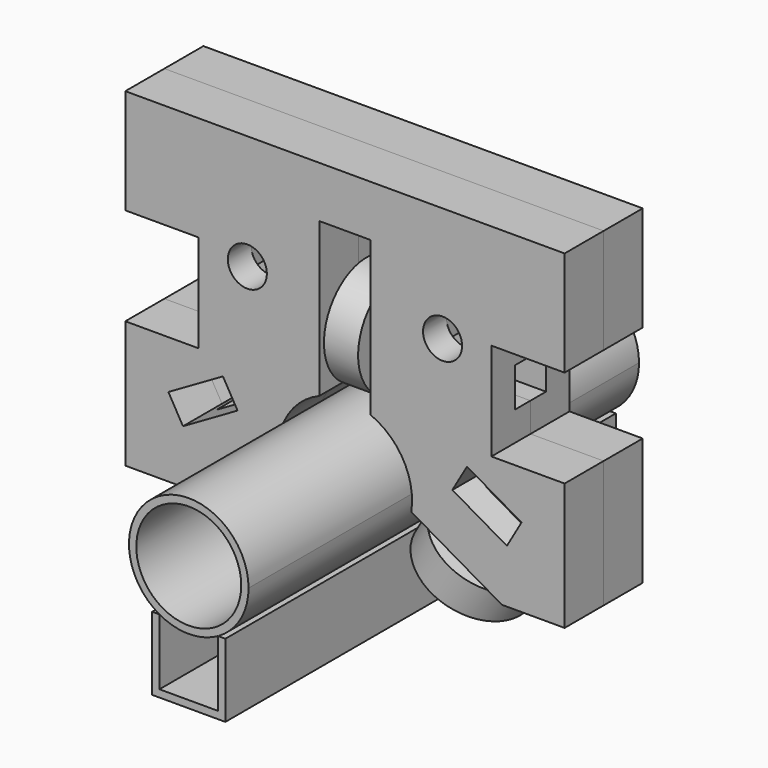
from build123d import *

# Parameters (mm, degrees)
F1_DEPTH = 50
F0_R     = 10.75
F2_R     = 11
F2_R_2   = 4
F3_DEPTH = 3.5
F5_COUNT = 3
F5_ANGLE = 240
F6_R     = 4
F7_DEPTH = 10
F9_DEPTH = 4


with BuildPart() as f1:
    # F0 (on Front) → F1 (new body, symmetric)
    with BuildSketch(Plane.XZ):
        Polygon((-6, -24.1800046816), (-6, -10.6800046816), (-7.5, -10.6800046816), (-7.5, -25.6800046816), (0, -25.6800046816), (7.5, -25.6800046816), (7.5, -10.6800046816), (6, -10.6800046816), (6, -24.1800046816), (0, -24.1800046816), align=None)
    extrude(amount=F1_DEPTH, both=True)


with BuildPart() as f1b:
    # F0 (on Front) → F1, piece 2 (new body, symmetric)
    with BuildSketch(Plane.XZ):
        with BuildLine():
            ThreePointArc((6, -10.6800046816), (10.5726652269, -6.1871843354), (12.25, 0))
            ThreePointArc((12.25, 0), (-6.1871843354, 10.5726652269), (-6, -10.6800046816))
            ThreePointArc((-6, -10.6800046816), (0, -12.25), (6, -10.6800046816))
        make_face()
        Circle(F0_R, mode=Mode.SUBTRACT)
    extrude(amount=F1_DEPTH, both=True)


with BuildPart() as f3:
    # F2 (on Right) → F3 (new body, symmetric)
    with BuildSketch(Plane.YZ):
        with Locations((0, 23.25)):
            Circle(F2_R)
        with Locations((0, 23.25)):
            Circle(F2_R_2, mode=Mode.SUBTRACT)
    extrude(amount=F3_DEPTH, both=True)


with BuildPart() as f5_1:
    # F5: instance of F3
    add(f3.part.rotate(Axis((0, 0, 0), (0, -1, 0)), 1 * F5_ANGLE / (F5_COUNT - 1)))


with BuildPart() as f5_2:
    # F5: instance of F3
    add(f3.part.rotate(Axis((0, 0, 0), (0, -1, 0)), 2 * F5_ANGLE / (F5_COUNT - 1)))


with BuildPart() as f7:
    # F6 (on Front) → F7 (new body)
    with BuildSketch(Plane.XZ):
        with BuildLine():
            ThreePointArc((5.25, 12.7082650271), (11.974631777, 6.7580096038), (13.5926495933, -2.0742172098))
            Line((13.5926495933, -2.0742172098), (32.1613700796, -12.7948729811))
            Line((32.1613700796, -12.7948729811), (45, -12.7948729811))
            Line((45, -12.7948729811), (45, 13.25))
            Line((45, 13.25), (30, 13.25))
            Line((30, 13.25), (30, 33.25))
            Line((30, 33.25), (45, 33.25))
            Line((45, 33.25), (45, 54.75))
            Line((45, 54.75), (0, 54.75))
            Line((0, 54.75), (-45, 54.75))
            Line((-45, 54.75), (-45, 33.25))
            Line((-45, 33.25), (-30, 33.25))
            Line((-30, 33.25), (-30, 13.25))
            Line((-30, 13.25), (-45, 13.25))
            Line((-45, 13.25), (-45, -12.7948729811))
            Line((-45, -12.7948729811), (-32.1613700796, -12.7948729811))
            Line((-32.1613700796, -12.7948729811), (-13.5926495933, -2.0742172098))
            ThreePointArc((-13.5926495933, -2.0742172098), (-11.974631777, 6.7580096038), (-5.25, 12.7082650271))
            Line((-5.25, 12.7082650271), (-5.25, 44.25))
            Line((-5.25, 44.25), (0, 44.25))
            Line((0, 44.25), (5.25, 44.25))
            Line((5.25, 44.25), (5.25, 12.7082650271))
        make_face()
        Polygon((-36.1776532222, 3.3615334795), (-25.0059255134, 9.8115334795), (-22.0059255134, 4.6153810568), (-33.1776532222, -1.8346189432), align=None, mode=Mode.SUBTRACT)
        Polygon((33.1776532222, -1.8346189432), (22.0059255134, 4.6153810568), (25.0059255134, 9.8115334795), (36.1776532222, 3.3615334795), align=None, mode=Mode.SUBTRACT)
        with Locations((-20, 31.25)):
            Circle(F6_R, mode=Mode.SUBTRACT)
        with Locations((20, 31.25)):
            Circle(F6_R, mode=Mode.SUBTRACT)
    extrude(amount=F7_DEPTH)

    # F8 (on face) → F9 (cut)
    with BuildSketch(Plane.XZ):
        Polygon((3.5, 27.25), (-3.5, 27.25), (-16, 27.25), (-20, 27.25), (-24, 27.25), (-45, 27.25), (-45, 19.25), (-3.5, 19.25), (3.5, 19.25), (45, 19.25), (45, 27.25), (24, 27.25), (20, 27.25), (16, 27.25), align=None)
        with BuildLine():
            Line((-20, 27.25), (-16, 27.25))
            Line((-16, 27.25), (-16, 31.25))
            ThreePointArc((-16, 31.25), (-17.1715728753, 28.4215728753), (-20, 27.25))
        make_face()
        with BuildLine():
            Line((16, 31.25), (16, 27.25))
            Line((16, 27.25), (20, 27.25))
            ThreePointArc((20, 27.25), (17.1715728753, 28.4215728753), (16, 31.25))
        make_face()
        with BuildLine():
            Line((-24, 27.25), (-20, 27.25))
            ThreePointArc((-20, 27.25), (-22.8284271247, 28.4215728753), (-24, 31.25))
            Line((-24, 31.25), (-24, 27.25))
        make_face()
        with BuildLine():
            ThreePointArc((-24, 31.25), (-22.8284271247, 28.4215728753), (-20, 27.25))
            ThreePointArc((-20, 27.25), (-17.1715728753, 28.4215728753), (-16, 31.25))
            ThreePointArc((-16, 31.25), (-20, 35.25), (-24, 31.25))
        make_face()
        with BuildLine():
            ThreePointArc((24, 31.25), (22.8284271247, 28.4215728753), (20, 27.25))
            Line((20, 27.25), (24, 27.25))
            Line((24, 27.25), (24, 31.25))
        make_face()
        with BuildLine():
            ThreePointArc((16, 31.25), (17.1715728753, 28.4215728753), (20, 27.25))
            ThreePointArc((20, 27.25), (22.8284271247, 28.4215728753), (24, 31.25))
            ThreePointArc((24, 31.25), (20, 35.25), (16, 31.25))
        make_face()
        Polygon((24.1709890229, 3.3653810568), (19.1709890229, -5.2948729811), (26.0991922531, -9.2948729811), (31.0991922531, -0.6346189432), align=None)
        Polygon((-19.1709890229, -5.2948729811), (-24.1709890229, 3.3653810568), (-31.0991922531, -0.6346189432), (-26.0991922531, -9.2948729811), align=None)
    extrude(amount=F9_DEPTH, mode=Mode.SUBTRACT)


with BuildPart() as f10_1:
    # F10: instance of F7
    add(f7.part.mirror(Plane(origin=(0, 0, 43.0121919212), x_dir=(-1, 0, 0), z_dir=(0, 1, 0))))


solid = Compound([f1.part, f1b.part, f3.part, f5_1.part, f5_2.part, f7.part, f10_1.part])
